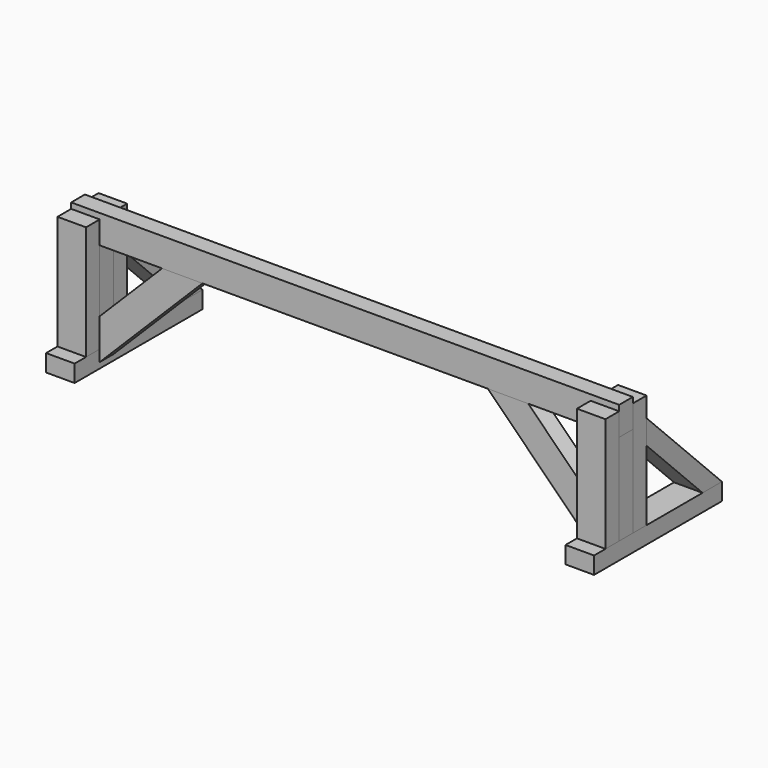
from build123d import *

# Parameters (mm, degrees)
F1_W      = 63.5
F1_H      = 355.6
F2_DEPTH  = 38.1
F3_W      = 63.5
F3_H      = 38.1
F4_DEPTH  = 203.2
F6_W      = 1219.2
F6_H      = 38.1
F7_DEPTH  = 63.5
F9_DEPTH  = 38.1
F11_W     = 63.5
F11_H     = 38.1
F12_DEPTH = 254
F15_DEPTH = 63.5


# Not quite as in the source:
# - a variable given as a bare number and used for a length is read in inches; the dataset says mm whatever the document's units were


with BuildPart() as f2:
    # F1 (on Top) → F2 (new body)
    with BuildSketch(Plane.XY):
        with Locations((-577.85, 76.2)):
            Rectangle(F1_W, F1_H)
    extrude(amount=F2_DEPTH)


with BuildPart() as f4:
    # F3 (on face) → F4 (new body)
    with BuildSketch(Plane.XY.offset(38.1)):
        with Locations((-577.85, -12.7)):
            Rectangle(F3_W, F3_H)
    extrude(amount=F4_DEPTH)


with BuildPart() as f5_1:
    # F5: instance of F4
    add(f4.part.mirror(Plane.YZ))


with BuildPart() as f5_2:
    # F5: instance of F2
    add(f2.part.mirror(Plane.YZ))


with BuildPart() as f7:
    # F6 (on face) → F7 (new body)
    with BuildSketch(Plane.XY.offset(241.3)):
        with Locations((0, -12.7)):
            Rectangle(F6_W, F6_H)
    extrude(amount=F7_DEPTH)


with BuildPart() as f9:
    # F8 (on face) → F9 (new body)
    with BuildSketch(Plane.XZ.offset(31.75)):
        Polygon((-407.3025612107, 241.3), (-546.1, 102.5025612107), (-546.1, 12.7), (-317.5, 241.3), align=None)
    extrude(amount=-F9_DEPTH)


with BuildPart() as f10_1:
    # F10: instance of F9
    add(f9.part.mirror(Plane.YZ))


with BuildPart() as f12:
    # F11 (on face) → F12 (new body)
    with BuildSketch(Plane.XY.offset(38.1)):
        with Locations((-577.85, -50.8)):
            Rectangle(F11_W, F11_H)
    extrude(amount=F12_DEPTH)


with BuildPart() as f12b:
    # F11 (on face) → F12, piece 2 (new body)
    with BuildSketch(Plane.XY.offset(38.1)):
        with Locations((-577.85, 25.4)):
            Rectangle(F11_W, F11_H)
    extrude(amount=F12_DEPTH)


with BuildPart() as f13_1:
    # F13: instance of F12b
    add(f12b.part.mirror(Plane.YZ))


with BuildPart() as f13_2:
    # F13: instance of F12
    add(f12.part.mirror(Plane.YZ))


with BuildPart() as f15:
    # F14 (on face) → F15 (new body)
    with BuildSketch(Plane.YZ.offset(609.6)):
        Polygon((44.45, 193.7684632736), (200.1184632736, 38.1), (254, 38.1), (44.45, 247.65), align=None)
    extrude(amount=-F15_DEPTH)


with BuildPart() as f16_1:
    # F16: instance of F15
    add(f15.part.mirror(Plane.YZ))


solid = Compound([f2.part, f4.part, f5_1.part, f5_2.part, f7.part, f9.part, f10_1.part, f12.part, f12b.part, f13_1.part, f13_2.part, f15.part, f16_1.part])
